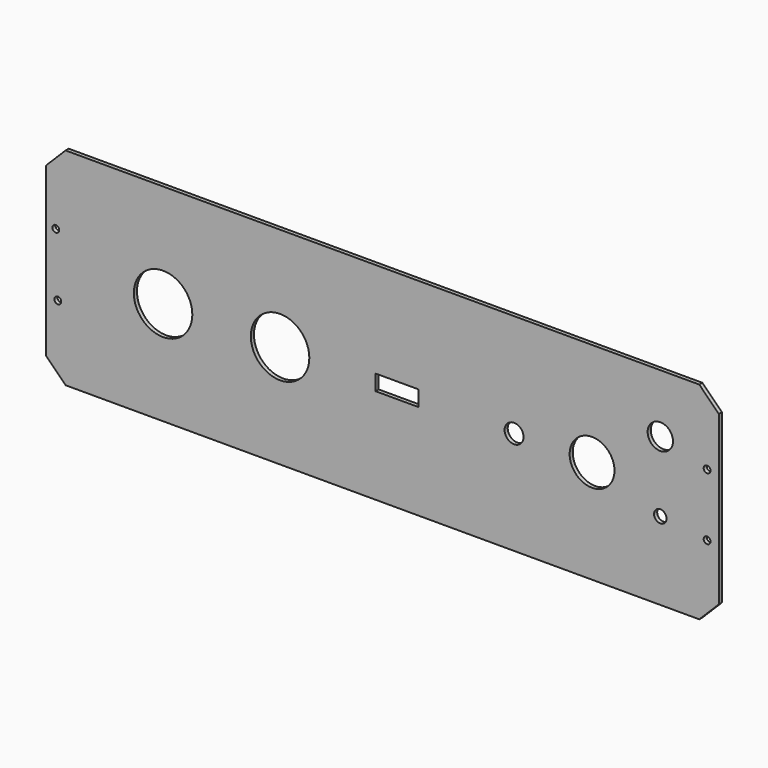
from build123d import *

# Parameters (mm, degrees)
F0_W      = 345
F0_H      = 106
F1_DEPTH  = 2
F2_SIZE   = 10
F3_SIZE   = 10
F4_R      = 1.75
F5_DEPTH  = 25
F6_R      = 15
F6_W      = 22
F6_H      = 8
F7_DEPTH  = 25
F9_R      = 6.5
F9_R_2    = 11.5
F9_R_3    = 3.2
F10_DEPTH = 25
F6_R_2    = 4.85
F11_DEPTH = 25


# Not quite as in the source:
# - a feature names something its author has since deleted; it is built from what else it names


with BuildPart() as f1:
    # F0 (on Front) → F1 (new body)
    with BuildSketch(Plane.XZ):
        with Locations((46.1619326359, 29.679378029)):
            Rectangle(F0_W, F0_H)
    extrude(amount=F1_DEPTH)

    # F2
    f2_edges = [f1.edges().sort_by_distance(p)[0] for p in [
        (-126.338067, -1, 82.679378),
    ]]
    chamfer(f2_edges, length=F2_SIZE)

    # F3
    f3_edges = [f1.edges().sort_by_distance(p)[0] for p in [
        (-126.338067, -1, -23.320622),
        (218.661933, -1, -23.320622),
        (218.661933, -1, 82.679378),
    ]]
    chamfer(f3_edges, length=F3_SIZE)

    # F4 (on face) → F5 (cut)
    with BuildSketch(Plane.XZ.offset(2)):
        with Locations((-121.3380673641, 45.679378029)):
            Circle(F4_R)
        with Locations((-120.3380673641, 13.679378029)):
            Circle(F4_R)
        with Locations((212.6619326359, 45.679378029)):
            Circle(F4_R)
        with Locations((212.6619326359, 13.679378029)):
            Circle(F4_R)
    extrude(amount=-F5_DEPTH, mode=Mode.SUBTRACT)

    # F6 (on face) → F7 (cut)
    with BuildSketch(Plane.XZ.offset(2)):
        with Locations((-66.3380673641, 29.679378029)):
            Circle(F6_R)
        with Locations((-6.3380673641, 29.679378029)):
            Circle(F6_R)
        with Locations((53.6619326359, 29.679378029)):
            Rectangle(F6_W, F6_H)
    extrude(amount=-F7_DEPTH, mode=Mode.SUBTRACT)

    # F9 (on face) → F10 (cut)
    with BuildSketch(Plane.XZ.offset(2)):
        with Locations((188.6619326359, 52.679378029)):
            Circle(F9_R)
        with Locations((153.6619326359, 29.679378029)):
            Circle(F9_R_2)
        with Locations((188.6619326359, 16.679378029)):
            Circle(F9_R_3)
    extrude(amount=-F10_DEPTH, mode=Mode.SUBTRACT)

    # F6 (on face) → F11 (cut)
    with BuildSketch(Plane.XZ.offset(2)):
        with Locations((-66.3380673641, 29.679378029)):
            Circle(F6_R)
        with Locations((-6.3380673641, 29.679378029)):
            Circle(F6_R)
        with Locations((53.6619326359, 29.679378029)):
            Rectangle(F6_W, F6_H)
        with Locations((113.6619326359, 29.679378029)):
            Circle(F6_R_2)
    extrude(amount=-F11_DEPTH, mode=Mode.SUBTRACT)


solid = f1.part
